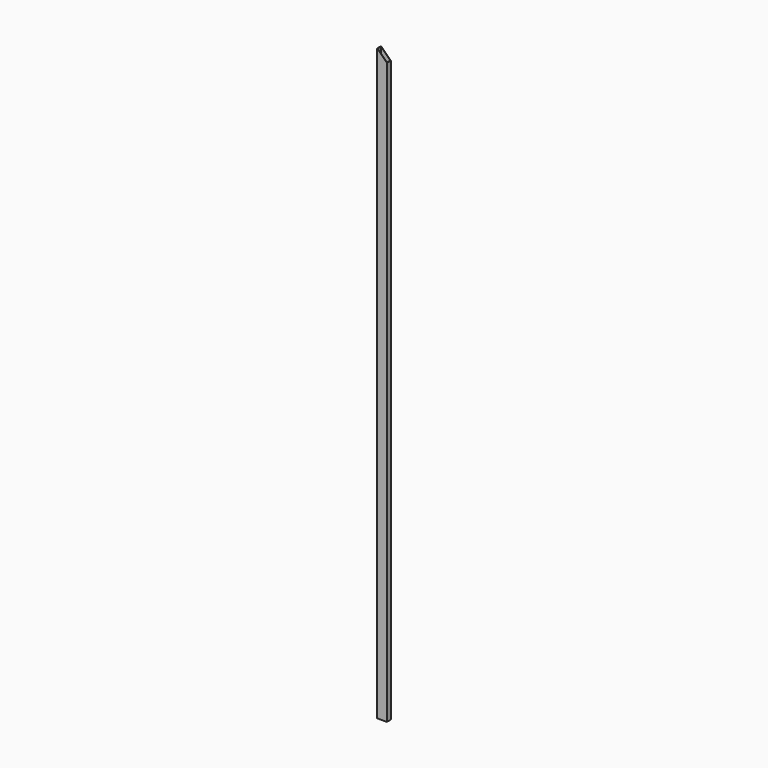
from build123d import *

# Parameters (mm, degrees)
F0_W        = 100
F0_H        = 50
F0_W_2      = 94
F0_H_2      = 44
F1_DEPTH    = 6070
F2_T1_DEPTH = 564.3365975932


# Not quite as in the source:
# - a fillet or chamfer that OpenCascade refuses, or shapes differently, is made with other operations: its cross-section is extruded or revolved along the edge and cut away or added


with BuildPart() as f1:
    # F0 (on Top) → F1 (new body)
    with BuildSketch(Plane.XY):
        with Locations((-3.195107216, 0)):
            Rectangle(F0_W, F0_H)
        with Locations((-3.195107216, 0)):
            Rectangle(F0_W_2, F0_H_2, mode=Mode.SUBTRACT)
    extrude(amount=F1_DEPTH)

    # F2: chamfer of 100 on 1 edges, made by hand

    # F2_s2 → F2_t1 (cut)
    with BuildSketch(Plane.XZ.offset(-282.1682987966)):
        Polygon((46.804892784, 5970), (-53.195107216, 6070), (46.804892784, 6070), align=None)
    extrude(amount=F2_T1_DEPTH, mode=Mode.SUBTRACT)


solid = f1.part
